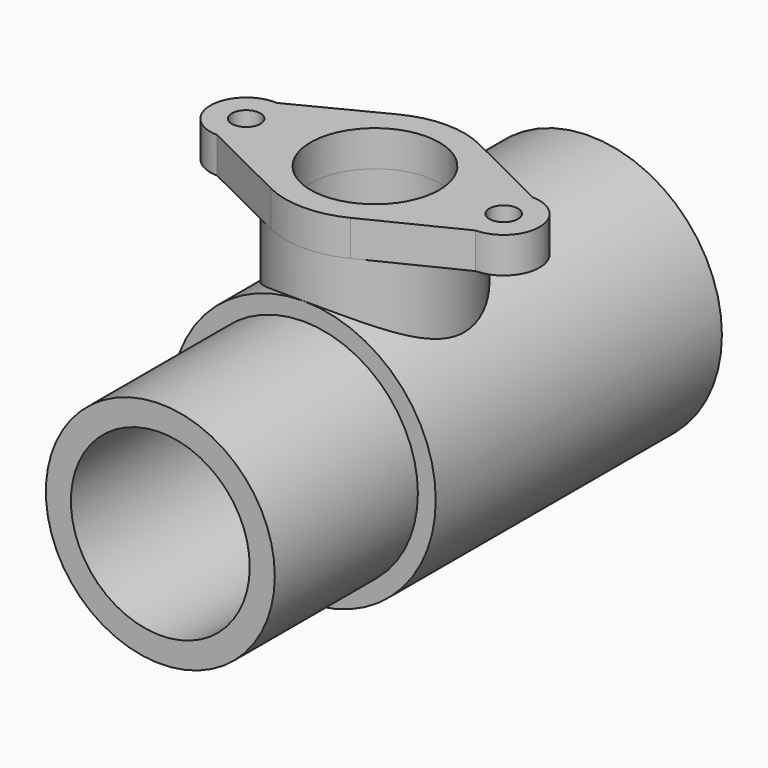
from build123d import *
from build123d import SkipClean  # not in build123d's __all__

# Parameters (mm, degrees)
F0_R        = 16
F0_R_2      = 12.5
F1_DEPTH    = 25
F0_R_3      = 18.5
F1_FACE_R   = 16
F1_FACE_R_2 = 12.5
F2_DEPTH    = 50
F3_R        = 16.1
F3_R_2      = 12.5
F4_DEPTH    = 25
F5_R        = 12.5
F5_R_2      = 9
F6_DEPTH    = 25
F7_R        = 12.5
F8_DEPTH    = 50
F9_R        = 9
F10_DEPTH   = 30
F11_R       = 2
F11_R_2     = 9
F12_DEPTH   = 5


with BuildPart() as f1:
    # F0 (on Front) → F1 (new body)
    with BuildSketch(Plane.XZ):
        Circle(F0_R)
        Circle(F0_R_2, mode=Mode.SUBTRACT)
    extrude(amount=F1_DEPTH)

    # F0 (on Front) + F1_face (on face) → F2 (join)
    with BuildSketch(Plane.XZ):
        Circle(F0_R_3)
        Circle(F0_R, mode=Mode.SUBTRACT)
    with BuildSketch(Plane(origin=(0, 0, 0), x_dir=(1, 0, 0), z_dir=(0, 1, 0))):
        Circle(F1_FACE_R)
        Circle(F1_FACE_R_2, mode=Mode.SUBTRACT)
    extrude(amount=-F2_DEPTH, dir=(0, -1, 0))

    # F3 (on face) → F4 (cut)
    with BuildSketch(Plane(origin=(0, 50, 0), x_dir=(-1, 0, 0), z_dir=(0, 1, 0))):
        Circle(F3_R)
        Circle(F3_R_2, mode=Mode.SUBTRACT)
    extrude(amount=-F4_DEPTH, mode=Mode.SUBTRACT)

    # F5 (on Top) → F6 (join)
    with BuildSketch(Plane.XY):
        with Locations((0, 12.5)):
            Circle(F5_R)
        with Locations((0, 12.5)):
            Circle(F5_R_2, mode=Mode.SUBTRACT)
    with SkipClean():  # cleaning this boolean's faces spoils the solid; the shape is the same uncleaned
        extrude(amount=F6_DEPTH)

    # F7 (on Front) → F8 (cut, symmetric)
    with BuildSketch(Plane.XZ):
        Circle(F7_R)
    extrude(amount=F8_DEPTH, both=True, mode=Mode.SUBTRACT)

    # F9 (on face) → F10 (cut)
    with BuildSketch(Plane.XY.offset(25)):
        with Locations((0, 12.5)):
            Circle(F9_R)
    extrude(amount=-F10_DEPTH, mode=Mode.SUBTRACT)

    # F11 (on face) → F12 (join)
    with BuildSketch(Plane.XY.offset(25)):
        with BuildLine():
            ThreePointArc((-17.6959947362, 17.4907495228), (-22.9942752122, 12.693442876), (-18.0829390199, 7.5006879354))
            Line((-18.0829390199, 7.5006879354), (-5.5433185763, 1.2963568799))
            ThreePointArc((-5.5433185763, 1.2963568799), (-12.4997271327, 12.4174069736), (-5.6908861674, 23.6294121422))
            Line((-5.6908861674, 23.6294121422), (-17.6959947362, 17.4907495228))
        make_face()
        with Locations((-18, 12.5)):
            Circle(F11_R, mode=Mode.SUBTRACT)
        with BuildLine():
            ThreePointArc((-5.6908861674, 23.6294121422), (-12.4997271327, 12.4174069736), (-5.5433185763, 1.2963568799))
            ThreePointArc((-5.5433185763, 1.2963568799), (-0.00079176, 2.51e-08), (5.5418992363, 1.2956547333))
            ThreePointArc((5.5418992363, 1.2956547333), (10.6189392233, 5.9054469619), (12.5, 12.5))
            ThreePointArc((12.5, 12.5), (10.6189392233, 19.0945530381), (5.5418992363, 23.7043452667))
            ThreePointArc((5.5418992363, 23.7043452667), (-0.0833847689, 24.9997218761), (-5.6908861674, 23.6294121422))
        make_face()
        with Locations((0, 12.5)):
            Circle(F11_R_2, mode=Mode.SUBTRACT)
        with BuildLine():
            ThreePointArc((12.5, 12.5), (10.6189392233, 5.9054469619), (5.5418992363, 1.2956547333))
            Line((5.5418992363, 1.2956547333), (18.0870791853, 7.500758336))
            ThreePointArc((18.0870791853, 7.500758336), (23.0086746295, 12.5), (18.0870791853, 17.499241664))
            Line((18.0870791853, 17.499241664), (5.5418992363, 23.7043452667))
            ThreePointArc((5.5418992363, 23.7043452667), (10.6189392233, 19.0945530381), (12.5, 12.5))
        make_face()
        with Locations((18, 12.5)):
            Circle(F11_R, mode=Mode.SUBTRACT)
    extrude(amount=F12_DEPTH)


solid = f1.part
